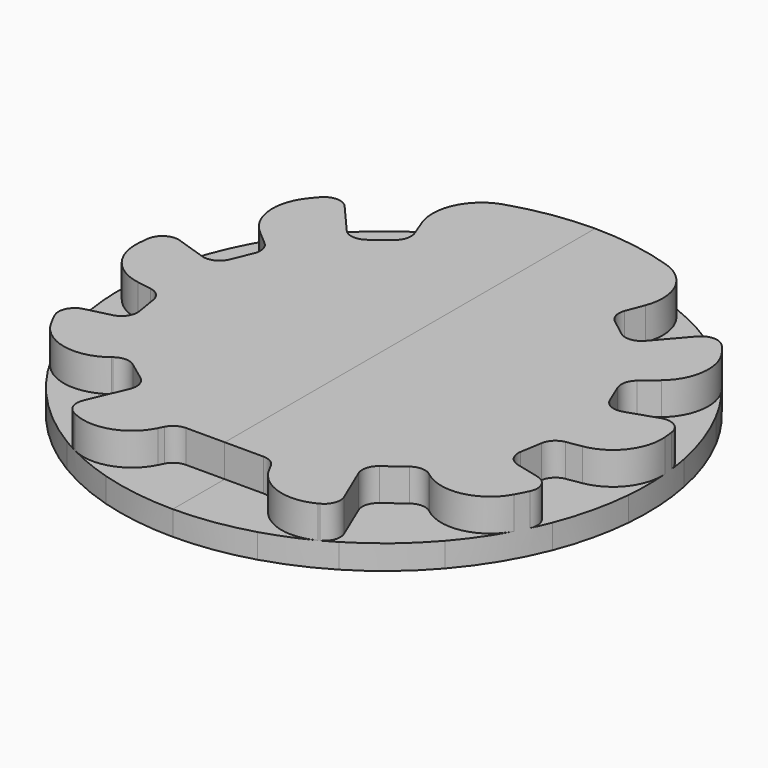
from build123d import *
from build123d import SkipClean  # not in build123d's __all__

# Parameters (mm, degrees)
F1_DEPTH    = 1.5
F2_DEPTH    = 3.5
F3_R        = 1
F4_R        = 1
F5_T1_DEPTH = 9.63963589
F5_T3_DEPTH = 10.6906794787
F5_T5_DEPTH = 9.0103178495
F5_T7_DEPTH = 9.246443515
F5_T9_DEPTH = 9.9071921997
F6_T1_DEPTH = 4.304276514
F6_T3_DEPTH = 5.0643678136
F6_T5_DEPTH = 5.03100669
F6_T7_DEPTH = 4.8959965939


# Not quite as in the source:
# - a fillet or chamfer that OpenCascade refuses, or shapes differently, is made with other operations: its cross-section is extruded or revolved along the edge and cut away or added
# - a feature names something its author has since deleted; it is built from what else it names


with BuildPart() as f1:
    # F0 (on Top) → F1 (new body)
    with BuildSketch(Plane.XY):
        with BuildLine():
            Line((0, -12.25), (0, -16.25))
            ThreePointArc((0, -16.25), (2.3542947693, -16.0785508097), (4.6589105316, -15.5678210633))
            Line((4.6589105316, -15.5678210633), (3, -12.25))
            Line((3, -12.25), (0, -12.25))
        make_face()
        with BuildLine():
            Line((3, -12.25), (4.6589105316, -15.5678210633))
            ThreePointArc((4.6589105316, -15.5678210633), (6.5703749152, -14.8624585272), (8.3785487777, -13.9234485807))
            Line((8.3785487777, -13.9234485807), (6.722135955, -10.0139320225))
            Line((6.722135955, -10.0139320225), (9.1300793123, -8.2245721403))
            Line((9.1300793123, -8.2245721403), (12.269716972, -10.6544143635))
            ThreePointArc((12.269716972, -10.6544143635), (13.901957351, -8.4141596021), (15.1297175637, -5.9290932226))
            Line((15.1297175637, -5.9290932226), (11.5782397372, -5.0612652418))
            Line((11.5782397372, -5.0612652418), (12.0646680977, -2.1009633231))
            Line((12.0646680977, -2.1009633231), (16.187616292, -1.4225254948))
            ThreePointArc((16.187616292, -1.4225254948), (16.2256082415, 0.890020895), (15.9349057476, 3.184537457))
            Line((15.9349057476, 3.184537457), (12.0646680977, 1.8990366769))
            Line((12.0646680977, 1.8990366769), (10.9139659303, 4.6695753469))
            Line((10.9139659303, 4.6695753469), (14.3535137791, 7.6183424833))
            ThreePointArc((14.3535137791, 7.6183424833), (13.1072409386, 9.6053492897), (11.5878961133, 11.3922413803))
            Line((11.5878961133, 11.3922413803), (8.5738108299, 7.9135966332))
            Line((8.5738108299, 7.9135966332), (6.2013811224, 9.7497821584))
            Line((6.2013811224, 9.7497821584), (7.9085498801, 14.1956802864))
            ThreePointArc((7.9085498801, 14.1956802864), (4.08550458, 15.7280371416), (0, 16.25))
            Line((0, 16.25), (0, -12.25))
            Line((0, -12.25), (3, -12.25))
        make_face()
        with BuildLine():
            Line((6.722135955, -10.0139320225), (8.3785487777, -13.9234485807))
            ThreePointArc((8.3785487777, -13.9234485807), (10.4527204974, -12.4419907653), (12.269716972, -10.6544143635))
            Line((12.269716972, -10.6544143635), (9.1300793123, -8.2245721403))
            Line((9.1300793123, -8.2245721403), (6.722135955, -10.0139320225))
        make_face()
        with BuildLine():
            ThreePointArc((11.5878961133, 11.3922413803), (9.8484856206, 12.9255495427), (7.9085498801, 14.1956802864))
            Line((7.9085498801, 14.1956802864), (6.2013811224, 9.7497821584))
            Line((6.2013811224, 9.7497821584), (8.5738108299, 7.9135966332))
            Line((8.5738108299, 7.9135966332), (11.5878961133, 11.3922413803))
        make_face()
        with BuildLine():
            Line((11.5782397372, -5.0612652418), (15.1297175637, -5.9290932226))
            ThreePointArc((15.1297175637, -5.9290932226), (15.8199601178, -3.7136722892), (16.187616292, -1.4225254948))
            Line((16.187616292, -1.4225254948), (12.0646680977, -2.1009633231))
            Line((12.0646680977, -2.1009633231), (11.5782397372, -5.0612652418))
        make_face()
        with BuildLine():
            ThreePointArc((15.9349057476, 3.184537457), (15.3056115889, 5.4590066762), (14.3535137791, 7.6183424833))
            Line((14.3535137791, 7.6183424833), (10.9139659303, 4.6695753469))
            Line((10.9139659303, 4.6695753469), (12.0646680977, 1.8990366769))
            Line((12.0646680977, 1.8990366769), (15.9349057476, 3.184537457))
        make_face()
    extrude(amount=F1_DEPTH)

    # F0 (on Top) → F2 (join)
    with BuildSketch(Plane.XY):
        with BuildLine():
            Line((3, -12.25), (4.6589105316, -15.5678210633))
            ThreePointArc((4.6589105316, -15.5678210633), (6.5703749152, -14.8624585272), (8.3785487777, -13.9234485807))
            Line((8.3785487777, -13.9234485807), (6.722135955, -10.0139320225))
            Line((6.722135955, -10.0139320225), (9.1300793123, -8.2245721403))
            Line((9.1300793123, -8.2245721403), (12.269716972, -10.6544143635))
            ThreePointArc((12.269716972, -10.6544143635), (13.901957351, -8.4141596021), (15.1297175637, -5.9290932226))
            Line((15.1297175637, -5.9290932226), (11.5782397372, -5.0612652418))
            Line((11.5782397372, -5.0612652418), (12.0646680977, -2.1009633231))
            Line((12.0646680977, -2.1009633231), (16.187616292, -1.4225254948))
            ThreePointArc((16.187616292, -1.4225254948), (16.2256082415, 0.890020895), (15.9349057476, 3.184537457))
            Line((15.9349057476, 3.184537457), (12.0646680977, 1.8990366769))
            Line((12.0646680977, 1.8990366769), (10.9139659303, 4.6695753469))
            Line((10.9139659303, 4.6695753469), (14.3535137791, 7.6183424833))
            ThreePointArc((14.3535137791, 7.6183424833), (13.1072409386, 9.6053492897), (11.5878961133, 11.3922413803))
            Line((11.5878961133, 11.3922413803), (8.5738108299, 7.9135966332))
            Line((8.5738108299, 7.9135966332), (6.2013811224, 9.7497821584))
            Line((6.2013811224, 9.7497821584), (7.9085498801, 14.1956802864))
            ThreePointArc((7.9085498801, 14.1956802864), (4.08550458, 15.7280371416), (0, 16.25))
            Line((0, 16.25), (0, -12.25))
            Line((0, -12.25), (3, -12.25))
        make_face()
    extrude(amount=F2_DEPTH)

    # F3
    f3_edges = [f1.edges().sort_by_distance(p)[0] for p in [
        (3, -12.25, 2.5),
        (9.130079, -8.224572, 2.5),
        (12.064668, -2.100963, 2.5),
        (10.913966, 4.669575, 2.5),
        (6.201381, 9.749782, 2.5),
    ]]
    fillet(f3_edges, radius=F3_R)

    # F4
    f4_edges = [f1.edges().sort_by_distance(p)[0] for p in [
        (12.064668, 1.899037, 2.5),
        (11.57824, -5.061265, 2.5),
        (6.722136, -10.013932, 2.5),
        (8.573811, 7.913597, 2.5),
    ]]
    fillet(f4_edges, radius=F4_R)

    # F5: fillet of radius 3 on 5 edges, made by hand

    # F5_s2 → F5_t1 (cut)
    with BuildSketch(Plane.XY.offset(1.5)):
        with BuildLine():
            ThreePointArc((7.4911310936, -14.4203139681), (5.1815062569, -14.6114030066), (3.4248714726, -13.0997429451))
            Line((3.4248714726, -13.0997429451), (4.6589105316, -15.5678210633))
            ThreePointArc((4.6589105316, -15.5678210633), (6.1020546546, -15.0607911144), (7.4911310936, -14.4203139681))
        make_face()
    extrude(amount=F5_T1_DEPTH, mode=Mode.SUBTRACT)

    # F5_s4 → F5_t3 (cut)
    with BuildSketch(Plane.XY.offset(1.5)):
        with BuildLine():
            ThreePointArc((14.2551270077, -7.800888026), (12.2362296702, -9.2974660849), (9.7872909338, -8.7332042566))
            Line((9.7872909338, -8.7332042566), (12.269716972, -10.6544143635))
            ThreePointArc((12.269716972, -10.6544143635), (13.3389463668, -9.2808948827), (14.2551270077, -7.800888026))
        make_face()
    extrude(amount=F5_T3_DEPTH, mode=Mode.SUBTRACT)

    # F5_s6 → F5_t5 (cut)
    with BuildSketch(Plane.XY.offset(1.5)):
        with BuildLine():
            ThreePointArc((16.1911606466, 1.381599405), (15.5696234502, -0.7158737175), (13.6891275029, -1.833655887))
            Line((13.6891275029, -1.833655887), (16.187616292, -1.4225254948))
            ThreePointArc((16.187616292, -1.4225254948), (16.2499870192, -0.0205396402), (16.1911606466, 1.381599405))
        make_face()
    extrude(amount=F5_T5_DEPTH, mode=Mode.SUBTRACT)

    # F5_s8 → F5_t7 (cut)
    with BuildSketch(Plane.XY.offset(1.5)):
        with BuildLine():
            ThreePointArc((12.7716701145, 10.0472355644), (13.3995013522, 7.899570062), (12.3664200817, 5.91478235))
            Line((12.3664200817, 5.91478235), (14.3535137791, 7.6183424833))
            ThreePointArc((14.3535137791, 7.6183424833), (13.6168564917, 8.8681294129), (12.7716701145, 10.0472355644))
        make_face()
    extrude(amount=F5_T7_DEPTH, mode=Mode.SUBTRACT)

    # F5_s10 → F5_t9 (cut)
    with BuildSketch(Plane.XY.offset(1.5)):
        with BuildLine():
            ThreePointArc((6.8847518154, 11.529451843), (6.7914209513, 13.8973561582), (5.0088339231, 15.4587865866))
            ThreePointArc((5.0088339231, 15.4587865866), (6.4894961639, 14.8979508503), (7.9085498801, 14.1956802864))
            Line((7.9085498801, 14.1956802864), (6.8847518154, 11.529451843))
        make_face()
    extrude(amount=F5_T9_DEPTH, mode=Mode.SUBTRACT)

    # F6: fillet of radius 1 on 4 edges, made by hand

    # F6_s2 → F6_t1 (cut)
    with BuildSketch(Plane.XY.offset(1.5)):
        with BuildLine():
            ThreePointArc((7.5756414815, -14.3760966936), (8.0513569254, -13.827282659), (8.0302135849, -13.1012971306))
            Line((8.0302135849, -13.1012971306), (8.3785487777, -13.9234485807))
            ThreePointArc((8.3785487777, -13.9234485807), (7.9803050872, -14.1554664605), (7.5756414815, -14.3760966936))
        make_face()
    extrude(amount=F6_T1_DEPTH, mode=Mode.SUBTRACT)

    # F6_s4 → F6_t3 (cut)
    with BuildSketch(Plane.XY.offset(1.5)):
        with BuildLine():
            ThreePointArc((14.6397584076, -7.0526572132), (14.6431333932, -6.1917144023), (13.9762230064, -5.6472289111))
            Line((13.9762230064, -5.6472289111), (15.1297175637, -5.9290932226))
            ThreePointArc((15.1297175637, -5.9290932226), (14.8953356428, -6.4954966006), (14.6397584076, -7.0526572132))
        make_face()
    extrude(amount=F6_T3_DEPTH, mode=Mode.SUBTRACT)

    # F6_s6 → F6_t5 (cut)
    with BuildSketch(Plane.XY.offset(1.5)):
        with BuildLine():
            ThreePointArc((16.1279854606, 1.9876078546), (15.6698492509, 2.7105535541), (14.82027687, 2.8143130881))
            Line((14.82027687, 2.8143130881), (15.9349057476, 3.184537457))
            ThreePointArc((15.9349057476, 3.184537457), (16.0426122647, 2.5878739778), (16.1279854606, 1.9876078546))
        make_face()
    extrude(amount=F6_T5_DEPTH, mode=Mode.SUBTRACT)

    # F6_s8 → F6_t7 (cut)
    with BuildSketch(Plane.XY.offset(1.5)):
        with BuildLine():
            ThreePointArc((10.8530428687, 10.544125571), (11.613004552, 10.8892780785), (12.3700450766, 10.5377646967))
            ThreePointArc((12.3700450766, 10.5377646967), (11.9865870504, 10.9719747942), (11.5878961133, 11.3922413803))
            Line((11.5878961133, 11.3922413803), (10.8530428687, 10.544125571))
        make_face()
    extrude(amount=F6_T7_DEPTH, mode=Mode.SUBTRACT)

    # F7: F1 across face


with BuildPart() as f1_1:
    add(f1.part, clean=False)
    with SkipClean():  # cleaning this boolean's faces spoils the solid; the shape is the same uncleaned
        add(f1.part.mirror(Plane(origin=(0, 1.0780141844, 1.6932624113), x_dir=(0, -1, 0), z_dir=(-1, 0, 0))), clean=False)


solid = f1_1.part
